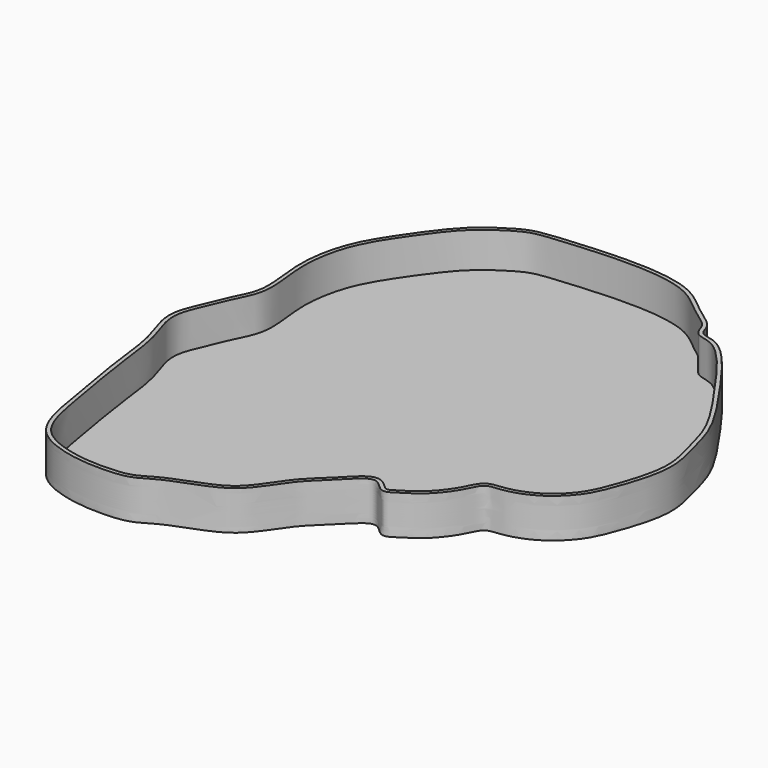
from build123d import *

# Parameters (mm, degrees)
F1_DEPTH = 10
F2_T     = -1


# Not quite as in the source:
# - the program builds the solid bodies; features that only make, move or delete a surface that nothing else refers to are left out


with BuildPart() as f1:
    # F0 (on Top) → F1 (new body)
    with BuildSketch(Plane.XY):
        with BuildLine():
            add(Edge.make_bspline(
                [(20.4343795776, 70.5794692039), (23.2255943634, 69.1610291324), (26.9729444714, 65.3586125558), (33.1115059027, 61.802307457), (33.353094905, 57.4243094852), (39.9485003526, 57.7829896142), (51.4564892401, 41.7209013553), (61.0042596604, 27.8371959959), (62.972342712, 18.8970400026), (66.0798432736, 8.9624596366), (61.8947210752, -3.9198011884), (58.7072826853, -11.5422109809), (51.7186085898, -17.6542399624), (44.6911757702, -19.6386799567), (40.557024863, -19.5231969213), (38.8946474266, -24.2693457111), (34.4352944942, -30.1768172802), (29.7615390973, -33.0351402567), (26.0155740701, -35.5913978153), (22.4451140773, -29.629090093), (16.0435216523, -37.287329721), (10.2958622914, -41.7471331624), (4.5252530384, -52.2716774174), (-4.2896512629, -55.6453750465), (-11.8448693641, -58.4991011379), (-16.2387565358, -61.7885708164), (-24.4672460338, -62.1636795067), (-32.0695741109, -61.5122745673), (-43.0272999465, -57.6681731042), (-45.8464268685, -46.377364224), (-46.7269967399, -39.6859611297), (-49.3113650115, -26.6210722433), (-50.5828375785, -13.2622323405), (-52.6903325787, -7.7122186299), (-54.717856371, -0.6963341265), (-50.8554992614, 6.9305449984), (-49.2148192971, 11.8800162074), (-45.248289308, 18.4507915844), (-48.1677997071, 30.7693982937), (-45.684423627, 43.9816988921), (-39.9588068391, 53.0972684254), (-32.255347465, 63.9370744348), (-26.323977847, 68.2282349033), (-21.3027434152, 71.3309022182), (-17.303654426, 72.1581748903), (-10.7112013183, 72.7883515104), (6.6565155143, 74.101399879), (16.8839318932, 72.3837363974), (20.4343795776, 70.5794692039)],
                knots=[0, 0, 0, 0, 0.0222021914, 0.0415321296, 0.0549624171, 0.0713770584, 0.10435517, 0.1358436241, 0.1580139281, 0.1818125087, 0.209051466, 0.2307977655, 0.2532198496, 0.273428668, 0.2873996682, 0.3031708528, 0.323731671, 0.3417105901, 0.3557641774, 0.3715349039, 0.3923655442, 0.4138156968, 0.4390217932, 0.4619996591, 0.4830787734, 0.500413361, 0.5212815544, 0.5425151912, 0.5670326547, 0.5913966084, 0.6111908214, 0.6386675756, 0.6662601616, 0.6844596541, 0.7040658002, 0.7255523705, 0.7428236383, 0.7626264276, 0.7889944813, 0.816245912, 0.8411591823, 0.8683045338, 0.8887621527, 0.9065222088, 0.9211594016, 0.9401421947, 0.9717586338, 1, 1, 1, 1], degree=3))
        make_face()
    extrude(amount=F1_DEPTH)

    # F2
    f2_openings = [f1.faces().sort_by_distance(p)[0] for p in [
        (0.157908, 9.12676, 10),
    ]]
    offset(amount=F2_T, openings=f2_openings)


solid = f1.part
